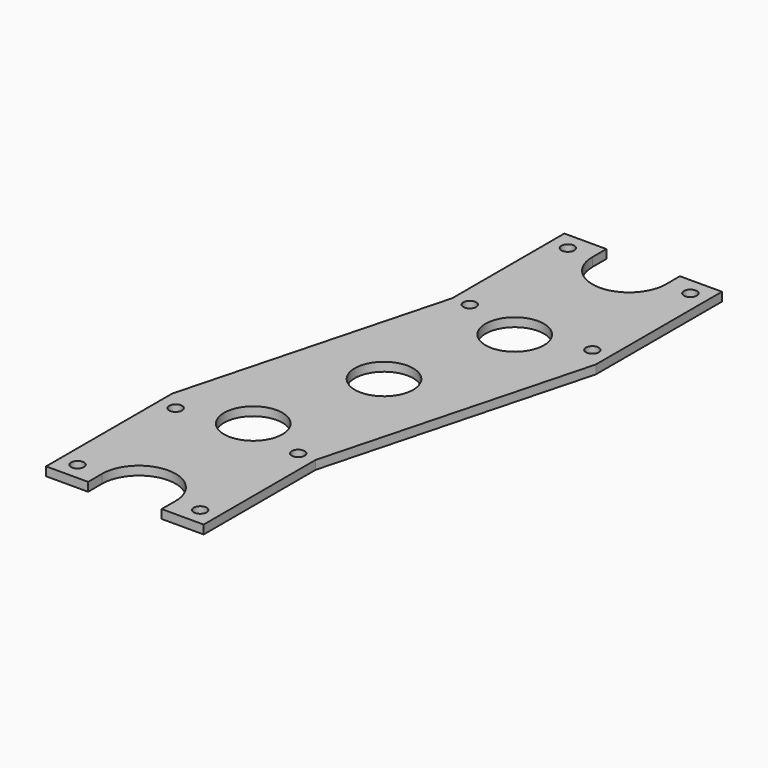
from build123d import *

# Parameters (mm, degrees)
F0_R     = 1.1
F1_DEPTH = 1.5
F2_W     = 12
F2_H     = 24
F3_DEPTH = 1.5
F4_R     = 5
F5_DEPTH = 1.5


# Not quite as in the source:
# - a feature names something its author has since deleted; it is built from what else it names


with BuildPart() as f1:
    # F0 (on Top) → F1 (new body)
    with BuildSketch(Plane.XY):
        with BuildLine():
            Line((-5.7, -48), (6.3, -48))
            Line((6.3, -48), (6.3, -45))
            ThreePointArc((6.3, -45), (0.9721111048, -38.7754518236), (-6, -43.0790627288))
            ThreePointArc((-6, -43.0790627288), (-5.7754518236, -44.0278888952), (-5.7, -45))
            Line((-5.7, -45), (-5.7, -48))
        make_face()
        with Locations((-1.5, -45)):
            Circle(F0_R, mode=Mode.SUBTRACT)
        with BuildLine():
            Line((25.5, -48), (25.5, 48))
            Line((25.5, 48), (6.3, 48))
            Line((6.3, 48), (6.3, 45))
            ThreePointArc((6.3, 45), (0, 38.7), (-6.3, 45))
            Line((-6.3, 45), (-6.3, 48))
            Line((-6.3, 48), (-25.5, 48))
            Line((-25.5, 48), (-25.5, -48))
            Line((-25.5, -48), (-18.3, -48))
            Line((-18.3, -48), (-18.3, -45))
            ThreePointArc((-18.3, -45), (-12.9721111048, -38.7754518236), (-6, -43.0790627288))
            ThreePointArc((-6, -43.0790627288), (0.9721111048, -38.7754518236), (6.3, -45))
            Line((6.3, -45), (6.3, -48))
            Line((6.3, -48), (25.5, -48))
        make_face()
        with Locations((-22.5, -45)):
            Circle(F0_R, mode=Mode.SUBTRACT)
        with Locations((-22.5, -24)):
            Circle(F0_R, mode=Mode.SUBTRACT)
        with Locations((-10.5, -24)):
            Circle(F0_R, mode=Mode.SUBTRACT)
        with Locations((-1.5, -24)):
            Circle(F0_R, mode=Mode.SUBTRACT)
        with Locations((10.5, -45)):
            Circle(F0_R, mode=Mode.SUBTRACT)
        with Locations((10.5, -24)):
            Circle(F0_R, mode=Mode.SUBTRACT)
        with Locations((-10.5, 24)):
            Circle(F0_R, mode=Mode.SUBTRACT)
        with Locations((-10.5, 45)):
            Circle(F0_R, mode=Mode.SUBTRACT)
        with Locations((10.5, 24)):
            Circle(F0_R, mode=Mode.SUBTRACT)
        with Locations((10.5, 45)):
            Circle(F0_R, mode=Mode.SUBTRACT)
        with Locations((-10.5, -24)):
            Circle(F0_R)
        with Locations((10.5, -45)):
            Circle(F0_R)
        with Locations((10.5, -24)):
            Circle(F0_R)
    extrude(amount=F1_DEPTH)

    # F2 (on face) → F3 (cut, through all)
    with BuildSketch(Plane(origin=(0, 0, 0), x_dir=(1, 0, 0), z_dir=(0, 0, -1))):
        Polygon((-13.5, -24), (-25.5, 21), (-25.5, -24), align=None)
        Polygon((25.5, 48), (13.5, 48), (13.5, 24), (13.5, -21), (13.5, -48), (25.5, -48), align=None)
        with Locations((-19.5, -36)):
            Rectangle(F2_W, F2_H)
        with Locations((7.5, 36)):
            Rectangle(F2_W, F2_H)
        Polygon((13.5, 24), (1.5, 24), (13.5, -21), align=None)
    extrude(amount=-F3_DEPTH, mode=Mode.SUBTRACT)

    # F4 (on face) → F5 (cut, through all)
    with BuildSketch(Plane(origin=(0, 0, 0), x_dir=(1, 0, 0), z_dir=(0, 0, -1))):
        with Locations((-0.4, -21)):
            Circle(F4_R)
        with Locations((-11.6, 21)):
            Circle(F4_R)
        with Locations((-6, 0)):
            Circle(F4_R)
    extrude(amount=-F5_DEPTH, mode=Mode.SUBTRACT)


solid = f1.part
